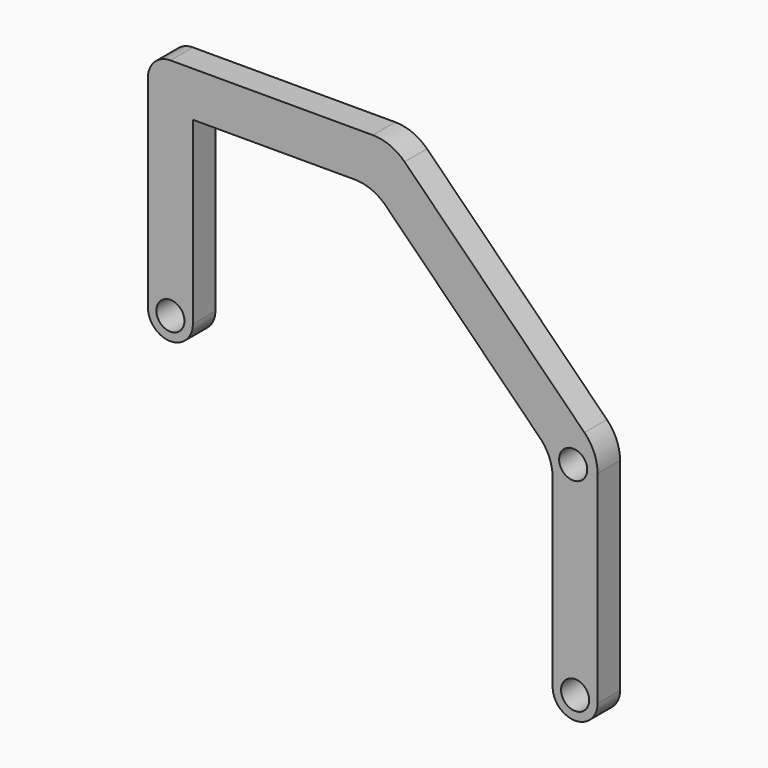
from build123d import *

# Parameters (mm, degrees)
F0_R     = 1.5875
F1_DEPTH = 3.175


# Not quite as in the source:
# - ends of sketch curves that miss each other by under 0.0002 mm in the source are joined
# - a feature names something its author has since deleted; it is built from what else it names


with BuildPart() as f1:
    # F0 (on Front) → F1 (new body)
    with BuildSketch(Plane.XZ):
        with BuildLine():
            Line((8.7026358494, -4.754912237), (7.4606623464, -3.512938734))
            ThreePointArc((7.4606623464, -3.512938734), (8.3275358886, -4.9102837361), (8.7026358494, -6.5113280243))
            Line((8.7026358494, -6.5113280243), (8.7026358494, -4.754912237))
        make_face()
        with BuildLine():
            Line((-10.3241423466, 14.271865959), (-11.6173641506, 15.565087763))
            Line((-11.6173641506, 15.565087763), (-13.4462559649, 15.565087763))
            ThreePointArc((-13.4462559649, 15.565087763), (-11.774512383, 15.185698369), (-10.3241423466, 14.271865959))
        make_face()
        with BuildLine():
            ThreePointArc((-8.0252617022, 19.1571902114), (-9.6733323142, 20.2583957881), (-11.6173641506, 20.645087763))
            Line((-11.6173641506, 20.645087763), (-11.6173641506, 15.565087763))
            Line((-11.6173641506, 15.565087763), (-8.0252617022, 19.1571902114))
        make_face()
        with BuildLine():
            ThreePointArc((13.7826358494, -4.7549120495), (13.3959438387, -2.810880314), (12.2947382978, -1.1628097886))
            Line((12.2947382978, -1.1628097886), (8.7026358494, -4.754912237))
            Line((8.7026358494, -4.754912237), (9.4338794152, -4.75491221))
            ThreePointArc((9.4338794152, -4.75491221), (11.0213794287, -3.167412237), (12.6088794152, -4.754912237))
            Line((12.6088794152, -4.754912237), (13.7826358494, -4.7549120495))
        make_face()
        with BuildLine():
            ThreePointArc((-34.4773641506, 20.645087763), (-36.2734153748, 19.9011389872), (-37.0173641506, 18.105087763))
            Line((-37.0173641506, 18.105087763), (-37.0173641506, -4.754912237))
            ThreePointArc((-37.0173641506, -4.754912237), (-34.4773641506, -7.294912237), (-31.9373641506, -4.754912237))
            Line((-31.9373641506, -4.754912237), (-31.9373641506, 13.025087763))
            Line((-31.9373641506, 13.025087763), (-31.9373641506, 15.565087763))
            Line((-31.9373641506, 15.565087763), (-31.9373641506, 20.645087763))
            Line((-31.9373641506, 20.645087763), (-34.4773641506, 20.645087763))
        make_face()
        with Locations((-34.4773641506, -4.754912237)):
            Circle(F0_R, mode=Mode.SUBTRACT)
        Polygon((-11.6173641506, 20.645087763), (-31.9373641506, 20.645087763), (-31.9373641506, 15.565087763), (-29.3973641506, 15.565087763), (-13.4462559649, 15.565087763), (-11.6173641506, 15.565087763), align=None)
        with BuildLine():
            ThreePointArc((11.2426358494, -30.154912237), (13.0386870736, -29.4109634612), (13.7826358494, -27.614912237))
            Line((13.7826358494, -27.614912237), (12.8301358494, -27.614912237))
            ThreePointArc((12.8301358494, -27.614912237), (11.2426358494, -29.202412237), (9.6551358494, -27.614912237))
            Line((9.6551358494, -27.614912237), (8.7026358494, -27.614912237))
            ThreePointArc((8.7026358494, -27.614912237), (9.4465846252, -29.4109634612), (11.2426358494, -30.154912237))
        make_face()
        with BuildLine():
            Line((9.4338794152, -4.75491221), (8.7026358494, -4.754912237))
            Line((8.7026358494, -4.754912237), (8.7026358494, -6.5113280243))
            Line((8.7026358494, -6.5113280243), (8.7026358494, -27.614912237))
            Line((8.7026358494, -27.614912237), (9.6551358494, -27.614912237))
            ThreePointArc((9.6551358494, -27.614912237), (11.2426358494, -26.027412237), (12.8301358494, -27.614912237))
            Line((12.8301358494, -27.614912237), (13.7826358494, -27.614912237))
            Line((13.7826358494, -27.614912237), (13.7826358494, -4.7549120495))
            Line((13.7826358494, -4.7549120495), (12.6088794152, -4.7549120928))
            ThreePointArc((12.6088794152, -4.7549120928), (11.0213794017, -6.342412237), (9.4338794152, -4.75491221))
        make_face()
        Polygon((-8.0252617022, 19.1571902114), (-11.6173641506, 15.565087763), (-10.3241423466, 14.271865959), (7.4606623464, -3.512938734), (8.7026358494, -4.754912237), (12.2947382978, -1.1628097886), align=None)
    extrude(amount=F1_DEPTH)


solid = f1.part
